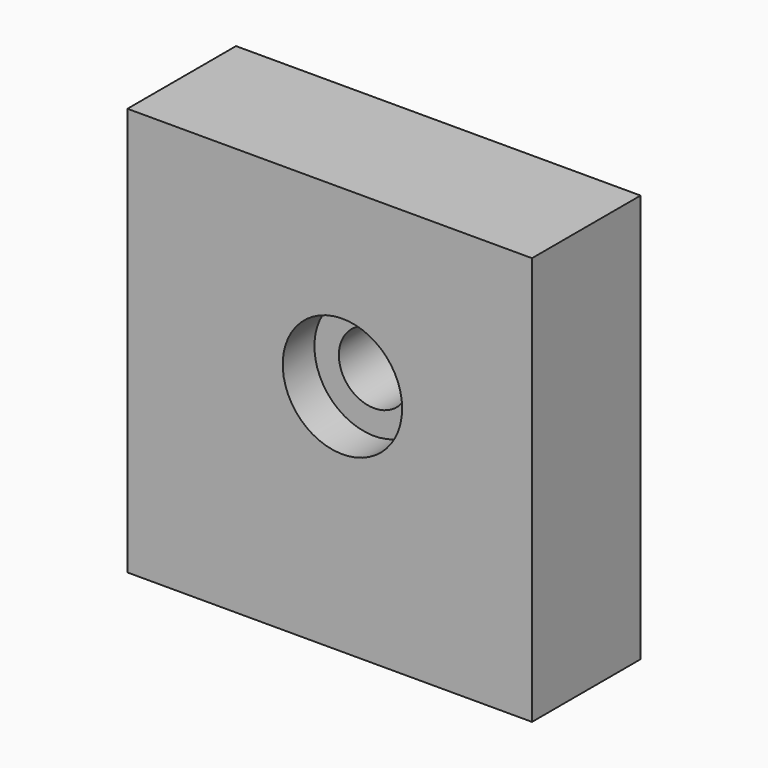
from build123d import *

# Parameters (mm, degrees)
F0_W           = 74.5297018439
F0_H           = 75.2062629908
F1_DEPTH       = 25
F6_D           = 13
F6_DEPTH       = 50
F6_CBORE_D     = 22
F6_CBORE_DEPTH = 7.3
F6_TIP         = 3.9055940237


# Not quite as in the source:
# - the program builds the solid bodies; features that only make, move or delete a surface that nothing else refers to are left out


with BuildPart() as f1:
    # F0 (on Front) → F1 (new body)
    with BuildSketch(Plane.XZ):
        with Locations((-55.4675785825, 15.8807532862)):
            Rectangle(F0_W, F0_H)
    extrude(amount=F1_DEPTH)

    # F6
    with Locations(Plane.XZ.offset(25)):
        with Locations((-53.1250275671, 21.3232878596)):
            CounterBoreHole(F6_D / 2, F6_CBORE_D / 2, F6_CBORE_DEPTH, depth=F6_DEPTH)
            with Locations((0, 0, -(F6_DEPTH + F6_TIP / 2))):  # 118° drill point
                Cone(0, F6_D / 2, F6_TIP, mode=Mode.SUBTRACT)


solid = f1.part
